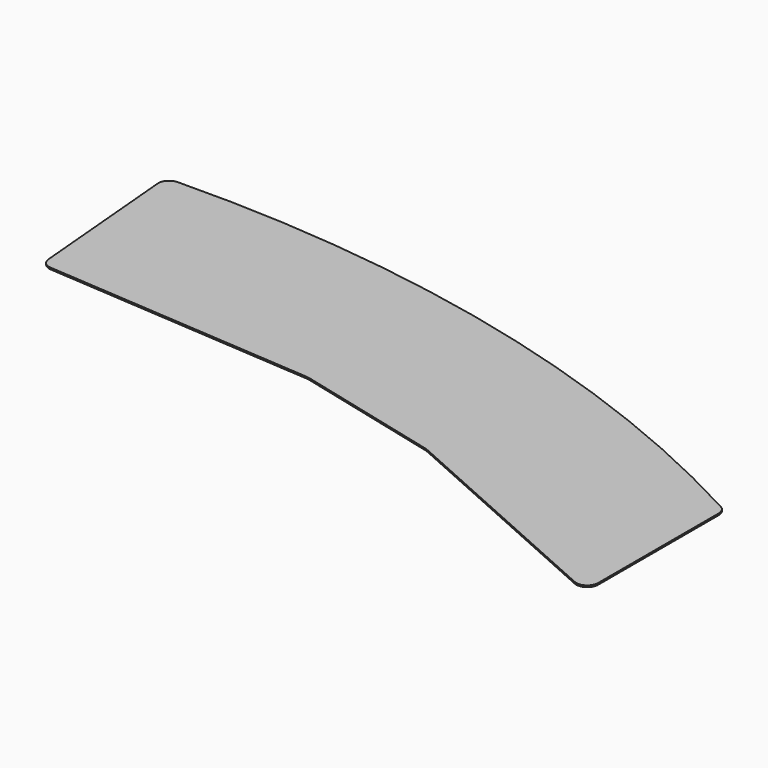
from build123d import *

# Parameters (mm, degrees)
F1_DEPTH = 1.5
F2_R     = 10
F3_R     = 20


with BuildPart() as f1:
    # F0 (on Top) → F1 (new body)
    with BuildSketch(Plane.XY):
        with BuildLine():
            Line((0, 36.5856099731), (0, 196.5856099731))
            ThreePointArc((0, 196.5856099731), (-307.3351576975, 315.2560594706), (-635, 349.5099039223))
            Line((-635, 349.5099039223), (-621.0269461922, 189.7971680702))
            Line((-621.0269461922, 189.7971680702), (-361.6779078132, 171.4103170113))
            Line((-361.6779078132, 171.4103170113), (-225.8692382849, 137.4102393502))
            Line((-225.8692382849, 137.4102393502), (0, 36.5856099731))
        make_face()
    extrude(amount=F1_DEPTH)

    # F2
    f2_edges = [f1.edges().sort_by_distance(p)[0] for p in [
        (0, 196.58561, 0.75),
        (-635, 349.509904, 0.75),
        (-621.026946, 189.797168, 0.75),
        (0, 36.58561, 0.75),
    ]]
    fillet(f2_edges, radius=F2_R)

    # F3
    f3_edges = [f1.edges().sort_by_distance(p)[0] for p in [
        (-361.677908, 171.410317, 0.75),
        (-225.869238, 137.410239, 0.75),
    ]]
    fillet(f3_edges, radius=F3_R)


solid = f1.part
